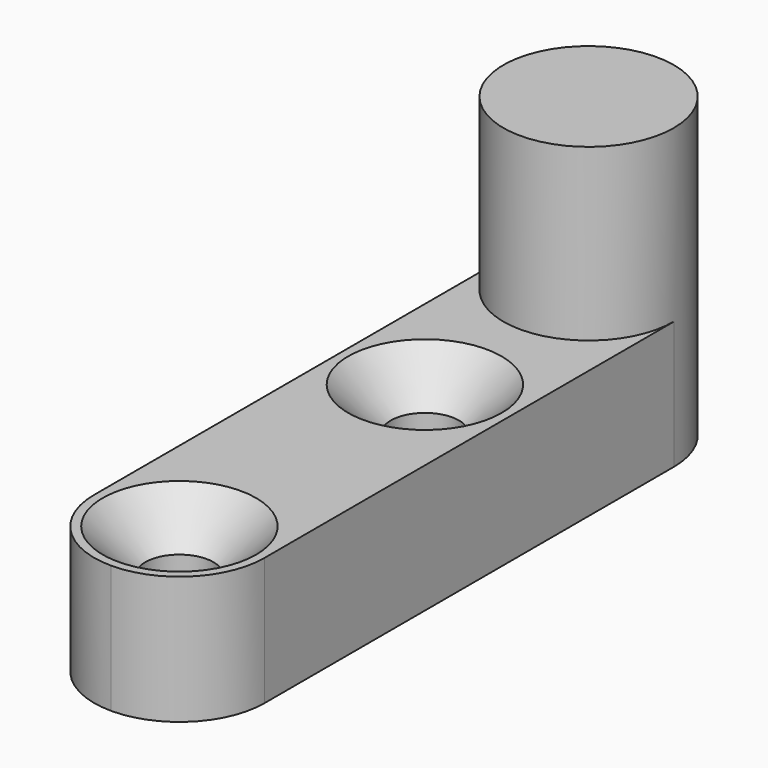
from build123d import *

# Parameters (mm, degrees)
F0_R     = 2
F1_DEPTH = 7.5
F2_DEPTH = 17.5
F3_SIZE2 = 2.5
F3_SIZE  = 2.5
F4_R     = 4.99999


# Not quite as in the source:
# - a fillet or chamfer is up to 0.001 mm smaller than in the source, because OpenCascade refuses the exact size


with BuildPart() as f1:
    # F0 (on Top) → F1 (new body)
    with BuildSketch(Plane.XY):
        with BuildLine():
            Line((5, -35), (5, 0))
            ThreePointArc((5, 0), (0, -5), (-5, 0))
            Line((-5, 0), (-5, -35))
            Line((-5, -35), (0, -35))
            Line((0, -35), (5, -35))
        make_face()
        with Locations((0, -30)):
            Circle(F0_R, mode=Mode.SUBTRACT)
        with Locations((0, -12)):
            Circle(F0_R, mode=Mode.SUBTRACT)
    extrude(amount=F1_DEPTH)

    # F0 (on Top) → F2 (join)
    with BuildSketch(Plane.XY):
        with BuildLine():
            ThreePointArc((-5, 0), (0, -5), (5, 0))
            ThreePointArc((5, 0), (0, 5), (-5, 0))
        make_face()
    extrude(amount=F2_DEPTH)

    # F3
    f3_edges = [f1.edges().sort_by_distance(p)[0] for p in [
        (-2, -12, 7.5),
        (-2, -30, 7.5),
    ]]
    chamfer(f3_edges, length=F3_SIZE, length2=F3_SIZE2)

    # F4 (radius 5 in the source; OpenCascade refuses exactly that, so slightly less here)
    f4_edges = [f1.edges().sort_by_distance(p)[0] for p in [
        (-5, -35, 3.75),
        (5, -35, 3.75),
    ]]
    fillet(f4_edges, radius=F4_R)


solid = f1.part
